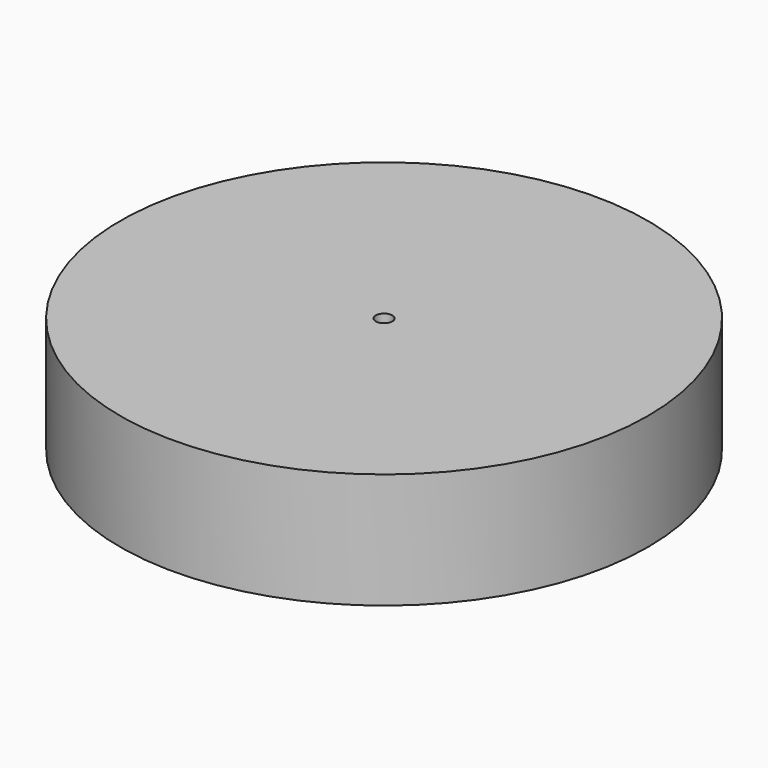
from build123d import *

# Parameters (mm, degrees)
F0_R     = 50.8
F0_R_2   = 1.5875
F1_DEPTH = 22.225


# Not quite as in the source:
# - a length typed as a fraction of an inch, garbled in the dataset ("3 / 203.2 mm" for 3/8 in), is restored


with BuildPart() as f1:
    # F0 (on Top) → F1 (new body)
    with BuildSketch(Plane.XY):
        Circle(F0_R)
        Circle(F0_R_2, mode=Mode.SUBTRACT)
    extrude(amount=F1_DEPTH)


solid = f1.part
